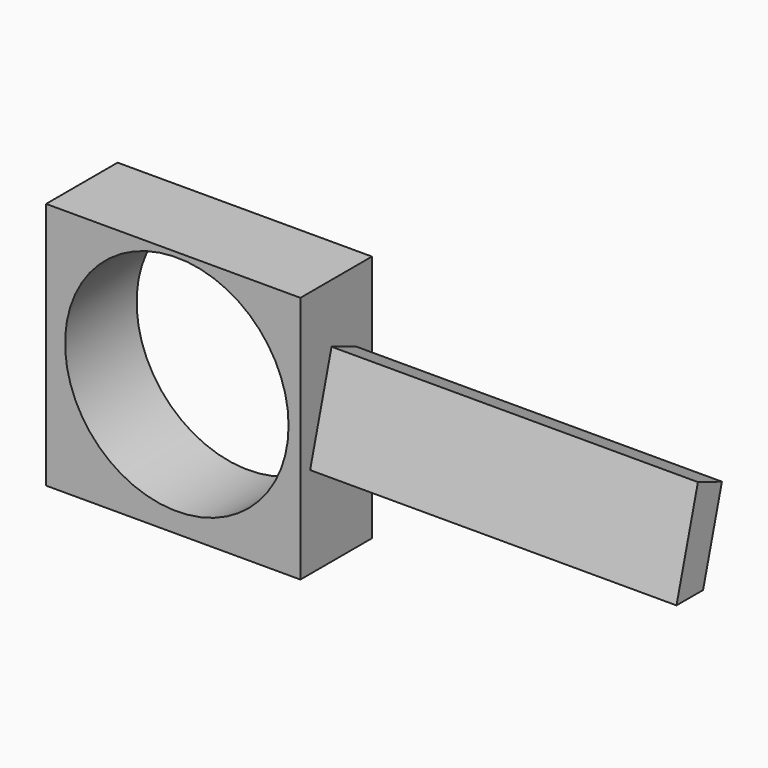
from build123d import *

# Parameters (mm, degrees)
F0_W     = 72.2630545497
F0_H     = 70.4785098787
F1_DEPTH = 25.4
F2_R     = 31.75
F3_DEPTH = 25.401
F5_DEPTH = 104.0980848


# Not quite as in the source:
# - an extrude ends at something that could not be found from the text; its depth is read off the source's solid


with BuildPart() as f1:
    # F0 (on Front) → F1 (new body)
    with BuildSketch(Plane.XZ):
        with Locations((36.1315272748, 34.5705245854)):
            Rectangle(F0_W, F0_H)
    extrude(amount=F1_DEPTH)

    # F2 (on face) → F3 (cut, through all)
    with BuildSketch(Plane.XZ.offset(25.4)):
        with Locations((37.1520854533, 36.7239564657)):
            Circle(F2_R)
    extrude(amount=-F3_DEPTH, mode=Mode.SUBTRACT)

    # F4 (on face) → F5 (join, through all)
    with BuildSketch(Plane.YZ.offset(72.2630545497)):
        Polygon((-12.5073632225, 25.324318558), (-5.8186161332, 49.7185699642), (-14.3406965322, 53.0769830369), (-21.9502989203, 25.324318558), align=None)
    extrude(amount=F5_DEPTH)


solid = f1.part
